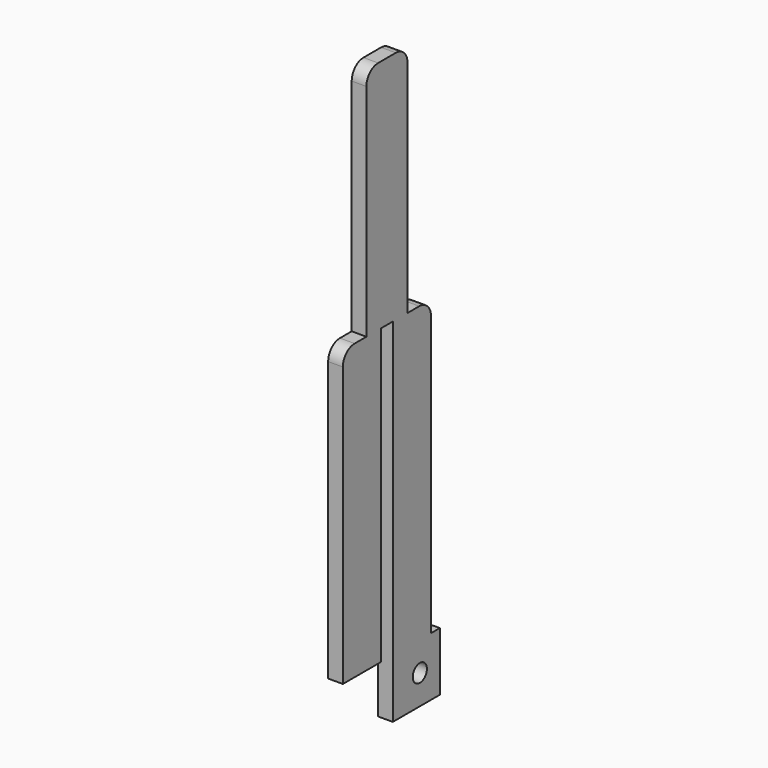
from build123d import *

# Parameters (mm, degrees)
F0_R     = 3.81
F1_DEPTH = 3.175


# Not quite as in the source:
# - ends of sketch curves that miss each other by under 0.0002 mm in the source are joined


with BuildPart() as f1:
    # F0 (on Right) → F1 (new body, symmetric)
    with BuildSketch(Plane.YZ):
        Polygon((28.575, -63.5), (23.8125, -63.5), (3.175, -63.5), (3.175, -88.9), (28.575, -88.9), align=None)
        with Locations((17.78, -76.2)):
            Circle(F0_R, mode=Mode.SUBTRACT)
        with BuildLine():
            Line((3.175, -63.5), (23.8125, -63.5))
            Line((23.8125, -63.5), (23.8125, 57.15))
            ThreePointArc((23.8125, 57.15), (21.9533763667, 61.6393796296), (17.4646167058, 63.4999996472))
            Line((17.4646167058, 63.4999996472), (17.4625, 63.5))
            Line((17.4625, 63.5), (11.1139111112, 63.5))
            Line((11.1139111112, 63.5), (11.124494366, 158.7492930333))
            ThreePointArc((11.124494366, 158.7492930333), (9.2648719104, 163.2398771909), (4.7744944052, 165.0999985889))
            Line((4.7744944052, 165.0999985889), (-4.7498, 165.0999985889))
            ThreePointArc((-4.7498, 165.0999985889), (-9.2399280605, 163.2401266494), (-11.0998, 158.7499985889))
            Line((-11.0998, 158.7499985889), (-11.0998, 63.5))
            Line((-11.0998, 63.5), (-17.4498, 63.5))
            Line((-17.4498, 63.5), (-17.4625, 63.5))
            ThreePointArc((-17.4625, 63.5), (-21.9526280605, 61.6401280605), (-23.8125, 57.15))
            Line((-23.8125, 57.15), (-23.8125, -63.5))
            Line((-23.8125, -63.5), (-3.175, -63.5))
            Line((-3.175, -63.5), (-3.175, 63.5))
            Line((-3.175, 63.5), (3.175, 63.5))
            Line((3.175, 63.5), (3.175, -63.5))
        make_face()
    extrude(amount=F1_DEPTH, both=True)


solid = f1.part
